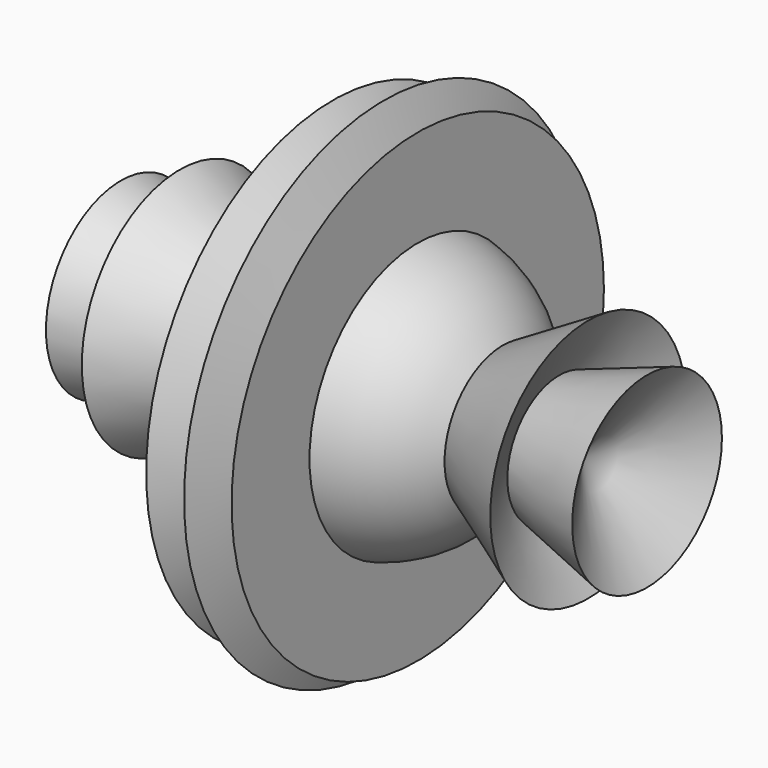
from build123d import *


# Not quite as in the source:
# - a feature names something its author has since deleted; it is built from what else it names


with BuildPart() as f1:
    # F0 (on Top) → F1 (revolve)
    with BuildSketch(Plane.XY):
        with BuildLine():
            Line((37.1953770518, 22.2900286317), (21.6585689027, 13.2690012092))
            ThreePointArc((21.6585689027, 13.2690012092), (15.0259859449, 20.4787633021), (6.1581879854, 24.6421736204))
            Line((6.1581879854, 24.6421736204), (6.1581879854, 42.3834808171))
            Line((6.1581879854, 42.3834808171), (3.0790939927, 36.7608899251))
            Line((3.0790939927, 36.7608899251), (0, 45.5001890659))
            Line((0, 45.5001890659), (-3.0941891787, 34.9035797321))
            Line((-3.0941891787, 34.9035797321), (-9.3218332717, 42.48192312))
            Line((-9.3218332717, 42.48192312), (-9.3218332717, 23.6275987873))
            ThreePointArc((-9.3218332717, 23.6275987873), (-16.3331401043, 19.4522115538), (-21.6585689027, 13.2690012092))
            Line((-21.6585689027, 13.2690012092), (-37.1953770518, 22.2900286317))
            Line((-37.1953770518, 22.2900286317), (-31.91267699, 11.7950700223))
            Line((-31.91267699, 11.7950700223), (-47.922976315, 17.042549327))
            Line((-47.922976315, 17.042549327), (-36.8364676833, 6.3755996525))
            Line((-36.8364676833, 6.3755996525), (-56.2179237604, 0))
            Line((-56.2179237604, 0), (36.3256136068, 0))
            Line((36.3256136068, 0), (47.922976315, 17.042549327))
            Line((47.922976315, 17.042549327), (31.91267699, 11.7950700223))
            Line((31.91267699, 11.7950700223), (37.1953770518, 22.2900286317))
        make_face()
    revolve(axis=Axis((-9.9461550768, 0, 0), (1, 0, 0)))


solid = f1.part
